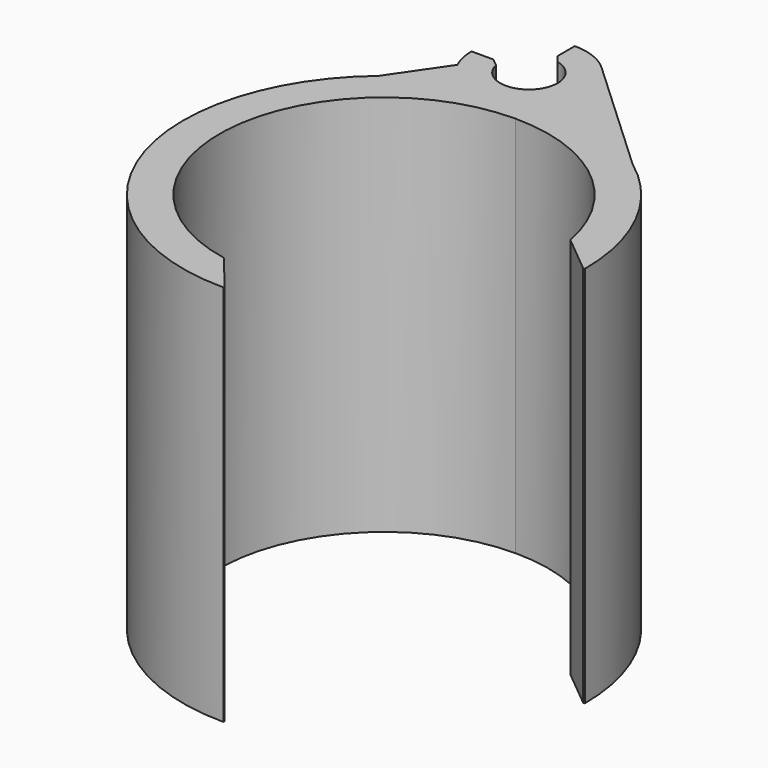
from build123d import *

# Parameters (mm, degrees)
F1_DEPTH    = 25.4
F3_DEPTH    = 25.4
F4_T1_DEPTH = 37.28706828
F5_T1_DEPTH = 27.7495122548


# Not quite as in the source:
# - a fillet or chamfer that OpenCascade refuses, or shapes differently, is made with other operations: its cross-section is extruded or revolved along the edge and cut away or added


with BuildPart() as f1:
    # F0 (on Top) → F1 (new body)
    with BuildSketch(Plane.XY):
        with BuildLine():
            ThreePointArc((0, 1.905), (1.3470384182, -1.3470384182), (-1.905, 0))
            Line((-1.905, 0), (-3.81, 0))
            ThreePointArc((-3.81, 0), (2.6940768363, -2.6940768363), (0, 3.81))
            Line((0, 3.81), (0, 1.905))
        make_face()
    extrude(amount=F1_DEPTH)

    # F2 (on face) → F3 (join)
    with BuildSketch(Plane.XY.offset(25.4)):
        with BuildLine():
            ThreePointArc((3.1994926084, -2.0686582726), (2.9633304397, -2.3947385463), (2.6940768363, -2.6940768363))
            Line((2.6940768363, -2.6940768363), (2.6940768363, -4.4720768363))
            ThreePointArc((2.6940768363, -4.4720768363), (10.4170971004, -7.6710565722), (13.6160768363, -15.3940768363))
            Line((13.6160768363, -15.3940768363), (16.0290768363, -15.3940768363))
            ThreePointArc((16.0290768363, -15.3940768363), (14.6027952108, -9.393689209), (10.6290540875, -4.6768775275))
            ThreePointArc((10.6290540875, -4.6768775275), (7.1111754901, -2.8118884542), (3.1994926084, -2.0686582726))
        make_face()
        with BuildLine():
            Line((2.5200781238, 2.8575), (2.6649185174, 2.7229229323))
            ThreePointArc((2.6649185174, 2.7229229323), (2.5933714137, 2.7911511444), (2.5200781238, 2.8575))
        make_face()
        with BuildLine():
            Line((2.6940768363, -4.4720768363), (2.6940768363, -2.6940768363))
            ThreePointArc((2.6940768363, -2.6940768363), (0.2570925649, -3.8013160107), (-2.3067877079, -3.0322978862))
            ThreePointArc((-2.3067877079, -3.0322978862), (-4.1681303207, -3.9602525446), (-5.862543163, -5.1663459449))
            ThreePointArc((-5.862543163, -5.1663459449), (-9.840056888, -19.9457487029), (2.6940768363, -28.7290768363))
            Line((2.6940768363, -28.7290768363), (2.6940768363, -26.3160768363))
            ThreePointArc((2.6940768363, -26.3160768363), (-8.2279231637, -15.3940768363), (2.6940768363, -4.4720768363))
        make_face()
        with BuildLine():
            ThreePointArc((2.6649185174, 2.7229229323), (3.7865078996, 0.4224428078), (3.1994926084, -2.0686582726))
            ThreePointArc((3.1994926084, -2.0686582726), (7.1111754901, -2.8118884542), (10.6290540875, -4.6768775275))
            Line((10.6290540875, -4.6768775275), (2.6649185174, 2.7229229323))
        make_face()
        with BuildLine():
            ThreePointArc((-5.862543163, -5.1663459449), (-4.1681303207, -3.9602525446), (-2.3067877079, -3.0322978862))
            ThreePointArc((-2.3067877079, -3.0322978862), (-2.9573260731, -2.4021495576), (-3.4407495541, -1.6362586916))
            Line((-3.4407495541, -1.6362586916), (-5.862543163, -5.1663459449))
        make_face()
    extrude(amount=-F3_DEPTH)

    # F4: chamfer of 2.54 on 2 edges, made by hand

    # F4_s2 → F4_t1 (cut)
    with BuildSketch(Plane.XY.offset(-5.94353414)):
        with BuildLine():
            Line((0.6333221193, -26.1199042634), (2.6940768363, -28.6142827349))
            Line((2.6940768363, -28.6142827349), (2.6940768363, -26.3160768363))
            ThreePointArc((2.6940768363, -26.3160768363), (1.6230071606, -26.2634325555), (0.6333221193, -26.1199042634))
        make_face()
        with BuildLine():
            Line((15.9142827349, -15.3940768363), (13.4199042634, -13.3333221193))
            ThreePointArc((13.4199042634, -13.3333221193), (13.5634325555, -14.3230071606), (13.6160768363, -15.3940768363))
            Line((13.6160768363, -15.3940768363), (15.9142827349, -15.3940768363))
        make_face()
    extrude(amount=F4_T1_DEPTH, mode=Mode.SUBTRACT)

    # F5: chamfer of 0.508 on 2 edges, made by hand

    # F5_s2 → F5_t1 (cut)
    with BuildSketch(Plane.XY.offset(-1.1747561274)):
        with BuildLine():
            Line((-1.8623055031, -0.4010526316), (-2.3589203039, 0))
            Line((-2.3589203039, 0), (-1.905, 0))
            ThreePointArc((-1.905, 0), (-1.8935148697, -0.2088694284), (-1.8623055031, -0.4010526316))
        make_face()
        with BuildLine():
            Line((0.4010526316, 1.8623055031), (0, 2.3589203039))
            Line((0, 2.3589203039), (0, 1.905))
            ThreePointArc((0, 1.905), (0.2088694284, 1.8935148697), (0.4010526316, 1.8623055031))
        make_face()
    extrude(amount=F5_T1_DEPTH, mode=Mode.SUBTRACT)


solid = f1.part
